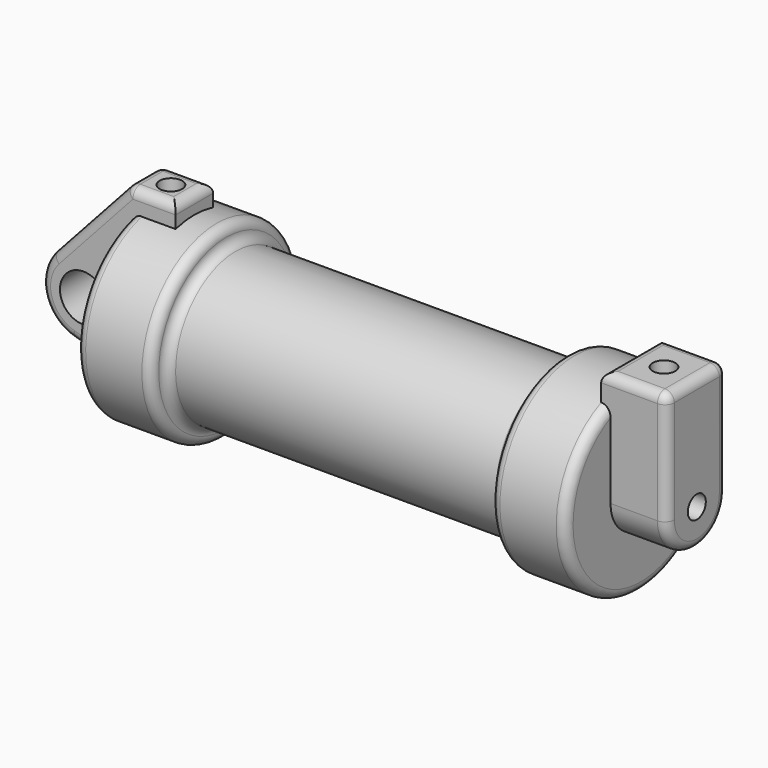
from build123d import *

# Parameters (mm, degrees)
F0_R      = 3.175
F1_DEPTH  = 3.175
F0_W      = 5.842
F0_H      = 12.7
F2_DEPTH  = 3.175
F4_R      = 1.524
F5_DEPTH  = 7.62
F6_DEPTH  = 1.27
F8_D      = 3.048
F8_DEPTH  = 10.414
F8_TIP    = 0.9157115834
F10_R     = 1.26999
F11_R     = 1.26999
F12_R     = 1.27
F13_R     = 1.27
F14_R     = 1.27
F14_2_R   = 1.27
F9_R      = 1.524
F15_DEPTH = 8.89


# Not quite as in the source:
# - a fillet or chamfer is up to 0.001 mm smaller than in the source, because OpenCascade refuses the exact size


with BuildPart() as f1:
    # F0 (on Front) → F1 (new body, symmetric)
    with BuildSketch(Plane.XZ):
        with BuildLine():
            Line((-0.9398, 0), (0, 0))
            Line((0, 0), (0, 12.7))
            Line((0, 12.7), (5.842, 12.7))
            Line((5.842, 12.7), (5.842, 15.24))
            Line((5.842, 15.24), (-0.508, 15.24))
            Line((-0.508, 15.24), (-10.8806298187, 3.8475430269))
            ThreePointArc((-10.8806298187, 3.8475430269), (-4.5919612295, 5.3297205562), (-0.9398, 0))
        make_face()
        with BuildLine():
            ThreePointArc((-8.1826630726, -5.5069827884), (-3.1957909266, -4.5493385486), (-0.9398, 0))
            ThreePointArc((-0.9398, 0), (-4.5919612295, 5.3297205562), (-10.8806298187, 3.8475430269))
            ThreePointArc((-10.8806298187, 3.8475430269), (-12.1459778134, -1.5837270034), (-8.1826630726, -5.5069827884))
        make_face()
        with Locations((-6.6548, 0)):
            Circle(F0_R, mode=Mode.SUBTRACT)
        with BuildLine():
            Line((5.842, 0), (0, 0))
            Line((0, 0), (-0.9398, 0))
            ThreePointArc((-0.9398, 0), (-3.1957909266, -4.5493385486), (-8.1826630726, -5.5069827884))
            Line((-8.1826630726, -5.5069827884), (5.842, -9.398))
            Line((5.842, -9.398), (5.842, 0))
        make_face()
    extrude(amount=F1_DEPTH, both=True)

    # F0 (on Front) → F2 (join, symmetric)
    with BuildSketch(Plane.XZ):
        with Locations((2.921, 6.35)):
            Rectangle(F0_W, F0_H)
    extrude(amount=F2_DEPTH, both=True)

    # F14
    f14_edges = [f1.edges().sort_by_distance(p)[0] for p in [
        (5.842, 0, 15.24),
        (2.667, -3.175, 15.24),
        (-0.508, 0, 15.24),
        (2.667, 3.175, 15.24),
        (-5.694315, -3.175, 9.543772),
        (-5.694315, 3.175, 9.543772),
    ]]
    fillet(f14_edges, radius=F14_R)


with BuildPart() as f3:
    # F0 (on Front) → F3 (revolve)
    with BuildSketch(Plane.XZ):
        Polygon((5.842, 12.7), (5.842, 0), (66.294, 0), (66.294, 12.7), (56.134, 12.7), (56.134, 10.16), (10.16, 10.16), (10.16, 12.7), align=None)
        with Locations((2.921, 6.35)):
            Rectangle(F0_W, F0_H)
    revolve(axis=Axis((33.147, 0, 0), (-1, 0, 0)))

    # F4 (on face) → F5 (join)
    with BuildSketch(Plane.YZ.offset(66.294)):
        with BuildLine():
            ThreePointArc((-5.08, 0), (0, -5.08), (5.08, 0))
            ThreePointArc((5.08, 0), (0, 5.08), (-5.08, 0))
        make_face()
        Circle(F4_R, mode=Mode.SUBTRACT)
        with BuildLine():
            ThreePointArc((-5.08, 0), (0, 5.08), (5.08, 0))
            Line((5.08, 0), (5.08, 15.24))
            Line((5.08, 15.24), (-5.08, 15.24))
            Line((-5.08, 15.24), (-5.08, 0))
        make_face()
    extrude(amount=F5_DEPTH)

    # F6 (add): a face of the model
    f6_faces = [f3.faces().sort_by_distance(p)[0] for p in [
        (66.294, 0, 13.7792682875),
    ]]
    extrude(f6_faces, amount=F6_DEPTH)

    # F8
    with Locations(Plane.XY.offset(15.24)):
        with Locations((69.469, 0)):
            Hole(F8_D / 2, depth=F8_DEPTH)
            with Locations((0, 0, -(F8_DEPTH + F8_TIP / 2))):  # 118° drill point
                Cone(0, F8_D / 2, F8_TIP, mode=Mode.SUBTRACT)

    # F10 (radius 1.27 in the source; OpenCascade refuses exactly that, so slightly less here)
    f10_edges = [f3.edges().sort_by_distance(p)[0] for p in [
        (56.134, 0, -12.7),
        (56.134, 0, -10.16),
    ]]
    fillet(f10_edges, radius=F10_R)

    # F11 (radius 1.27 in the source; OpenCascade refuses exactly that, so slightly less here)
    f11_edges = [f3.edges().sort_by_distance(p)[0] for p in [
        (10.16, 0, -10.16),
        (10.16, 0, -12.7),
    ]]
    fillet(f11_edges, radius=F11_R)

    # F12
    f12_edges = [f3.edges().sort_by_distance(p)[0] for p in [
        (0, 0, -12.7),
    ]]
    fillet(f12_edges, radius=F12_R)

    # F13
    f13_edges = [f3.edges().sort_by_distance(p)[0] for p in [
        (66.294, 0, -12.7),
    ]]
    fillet(f13_edges, radius=F13_R)

    # F14#2
    f14_2_edges = [f3.edges().sort_by_distance(p)[0] for p in [
        (73.914, -5.08, 7.62),
        (69.469, -5.08, 15.24),
        (69.469, 5.08, 15.24),
        (73.914, 0, 15.24),
        (65.024, 0, 15.24),
    ]]
    fillet(f14_2_edges, radius=F14_2_R)


with BuildPart() as f15_tool:
    # F9 (on face) → F15 (new body, symmetric)
    with BuildSketch(Plane.XY.offset(15.24)):
        with Locations((2.667, 0)):
            Circle(F9_R)
    extrude(amount=F15_DEPTH, both=True)


with BuildPart() as f1_1:
    add(f1.part)

    # F15: cut by f15_tool
    add(f15_tool.part, mode=Mode.SUBTRACT)


with BuildPart() as f3_1:
    add(f3.part)

    # F15: cut by f15_tool
    add(f15_tool.part, mode=Mode.SUBTRACT)


solid = Compound([f1_1.part, f3_1.part])
